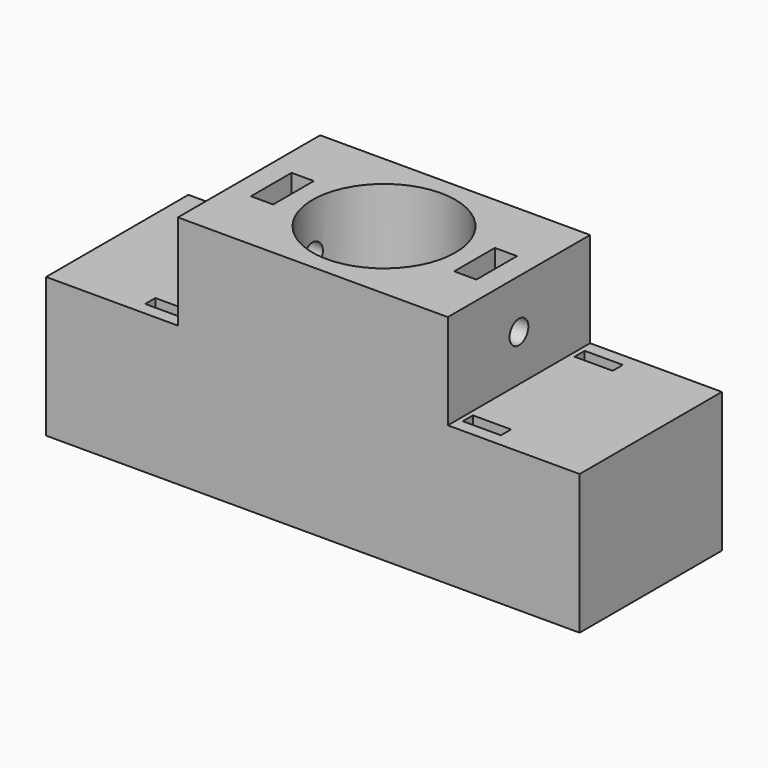
from build123d import *

# Parameters (mm, degrees)
F1_DEPTH  = 22
F3_R      = 11.25
F4_DEPTH  = 16
F5_DEPTH  = 18
F6_R      = 4.75
F7_DEPTH  = 4
F8_W      = 3
F8_H      = 2
F9_DEPTH  = 22
F11_DEPTH = 15
F12_R     = 11.25
F13_DEPTH = 15
F14_R     = 1.85
F15_DEPTH = 50.8
F17_DEPTH = 9.8


# Not quite as in the source:
# - a feature names something its author has since deleted; it is built from what else it names


with BuildPart() as f1:
    # F0 (on Top) → F1 (new body)
    with BuildSketch(Plane.XY):
        with BuildLine():
            ThreePointArc((1.21e-08, -14), (9.8994949409, -9.8994949323), (14, 0))
            ThreePointArc((14, 0), (9.8994949202, 9.899494953), (-4.65e-08, 14))
            ThreePointArc((-4.65e-08, 14), (-14, -2.93e-08), (1.21e-08, -14))
        make_face()
        with BuildLine():
            ThreePointArc((-4.65e-08, 14), (9.8994949202, 9.899494953), (14, 0))
            ThreePointArc((14, 0), (9.8994949409, -9.8994949323), (1.21e-08, -14))
            Line((1.21e-08, -14), (42, -14))
            Line((42, -14), (42, 14))
            Line((42, 14), (-4.65e-08, 14))
        make_face()
        with BuildLine():
            ThreePointArc((1.21e-08, -14), (-14, -2.93e-08), (-4.65e-08, 14))
            Line((-4.65e-08, 14), (-42, 14))
            Line((-42, 14), (-42, -14))
            Line((-42, -14), (1.21e-08, -14))
        make_face()
    extrude(amount=F1_DEPTH)

    # F3 (on face) → F4 (cut)
    with BuildSketch(Plane.XY.offset(22)):
        Circle(F3_R)
    extrude(amount=-F4_DEPTH, mode=Mode.SUBTRACT)

    # F2 (on face) → F5 (cut)
    with BuildSketch(Plane.XY.offset(22)):
        with BuildLine():
            Line((-6, 3.8887658711), (-6, -3.8887658711))
            ThreePointArc((-6, -3.8887658711), (0, -7.15), (6, -3.8887658711))
            Line((6, -3.8887658711), (6, 3.8887658711))
            ThreePointArc((6, 3.8887658711), (0, 7.15), (-6, 3.8887658711))
        make_face()
    extrude(amount=-F5_DEPTH, mode=Mode.SUBTRACT)

    # F6 (on face) → F7 (cut)
    with BuildSketch(Plane.XY.offset(4)):
        Circle(F6_R)
    extrude(amount=-F7_DEPTH, mode=Mode.SUBTRACT)

    # F8 (on face) → F9 (cut)
    with BuildSketch(Plane.XY.offset(22)):
        with Locations((-26.5, 11)):
            Rectangle(F8_W, F8_H)
        with Locations((-23.5, 11)):
            Rectangle(F8_W, F8_H)
        with Locations((-23.5, -11)):
            Rectangle(F8_W, F8_H)
        with Locations((-26.5, -11)):
            Rectangle(F8_W, F8_H)
        with Locations((23.5, 11)):
            Rectangle(F8_W, F8_H)
        with Locations((26.5, 11)):
            Rectangle(F8_W, F8_H)
        with Locations((26.5, -11)):
            Rectangle(F8_W, F8_H)
        with Locations((23.5, -11)):
            Rectangle(F8_W, F8_H)
    extrude(amount=-F9_DEPTH, mode=Mode.SUBTRACT)

    # F10 (on face) → F11 (join)
    with BuildSketch(Plane.XY.offset(22)):
        Polygon((-21.25, -14), (21.25, -14), (21.25, 0), (21.25, 14), (-21.25, 14), align=None)
    extrude(amount=F11_DEPTH)

    # F12 (on face) → F13 (cut)
    with BuildSketch(Plane.XY.offset(37)):
        Circle(F12_R)
    extrude(amount=-F13_DEPTH, mode=Mode.SUBTRACT)

    # F14 (on face) → F15 (cut)
    with BuildSketch(Plane.YZ.offset(21.25)):
        with Locations((0, 29.2573869228)):
            Circle(F14_R)
    extrude(amount=-F15_DEPTH, mode=Mode.SUBTRACT)

    # F16 (on face) → F17 (cut)
    with BuildSketch(Plane.XY.offset(37)):
        Polygon((-14.25, -4), (-14.25, 4), (-17.75, 4), (-17.75, 1.1981789721), (-17.75, -4), align=None)
        Polygon((14.25, -4), (17.75, -4), (17.75, 0), (17.75, 4), (14.25, 4), align=None)
    extrude(amount=-F17_DEPTH, mode=Mode.SUBTRACT)


solid = f1.part
